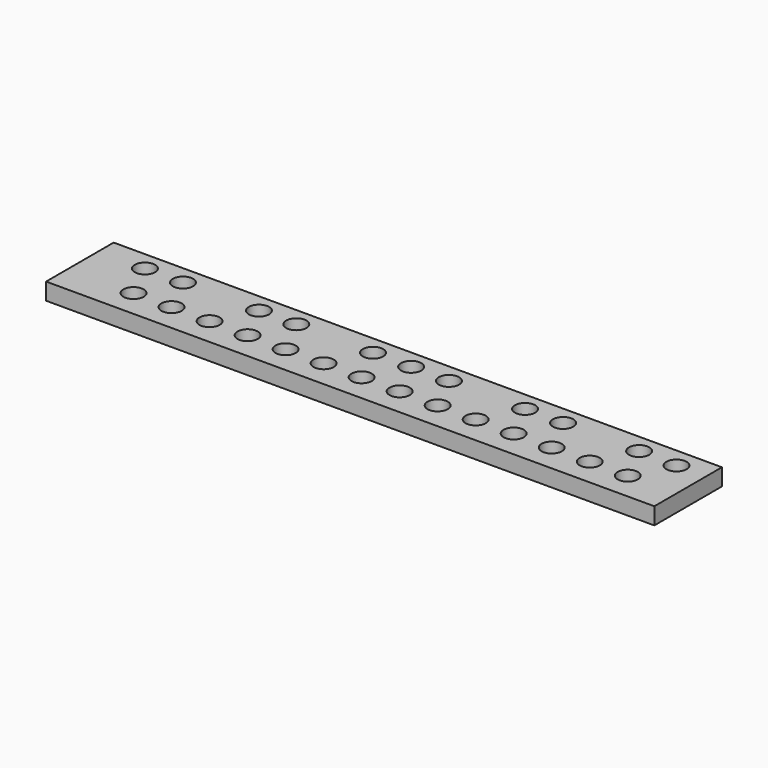
from build123d import *

# Parameters (mm, degrees)
F0_W     = 254
F0_H     = 50.8
F1_DEPTH = 1828.7999629974
F2_R     = 30.48
F3_DEPTH = 127


# Not quite as in the source:
# - a feature names something its author has since deleted; it is built from what else it names


with BuildPart() as f1:
    # F0 (on Right) → F1 (new body)
    with BuildSketch(Plane.YZ):
        with Locations((-10.6218170047, -93.1090038955)):
            Rectangle(F0_W, F0_H)
    extrude(amount=F1_DEPTH)

    # F2 (on Top) → F3 (cut)
    with BuildSketch(Plane.XY):
        with Locations((139.7, 59.2281829953)):
            Circle(F2_R)
        with Locations((254, 59.2281829953)):
            Circle(F2_R)
        with Locations((196.9066466086, -55.0718170047)):
            Circle(F2_R)
        with Locations((311.2066466086, -55.0718170047)):
            Circle(F2_R)
        with Locations((425.5066466086, -55.0718170047)):
            Circle(F2_R)
        with Locations((539.8066466086, -55.0718170047)):
            Circle(F2_R)
        with Locations((482.6, 59.2281829953)):
            Circle(F2_R)
        with Locations((594.391644001, 59.8655641079)):
            Circle(F2_R)
        with Locations((654.1066466086, -55.0718170047)):
            Circle(F2_R)
        with Locations((768.4066466086, -55.0718170047)):
            Circle(F2_R)
        with Locations((882.7066466086, -55.0718170047)):
            Circle(F2_R)
        with Locations((825.5, 59.2281829953)):
            Circle(F2_R)
        with Locations((940.1113390923, 59.2281829953)):
            Circle(F2_R)
        with Locations((997.0066466086, -55.0718170047)):
            Circle(F2_R)
        with Locations((1111.3066466086, -55.0718170047)):
            Circle(F2_R)
        with Locations((1054.1, 58.8000789285)):
            Circle(F2_R)
        with Locations((1225.6066466086, -55.0718170047)):
            Circle(F2_R)
        with Locations((1339.9066466086, -55.0718170047)):
            Circle(F2_R)
        with Locations((1282.7, 59.2281829953)):
            Circle(F2_R)
        with Locations((1397, 59.2281829953)):
            Circle(F2_R)
        with Locations((1454.2066466086, -55.0718170047)):
            Circle(F2_R)
        with Locations((1568.5066466086, -55.0718170047)):
            Circle(F2_R)
        with Locations((1625.6, 59.2281829953)):
            Circle(F2_R)
        with Locations((1682.8066466086, -55.0718170047)):
            Circle(F2_R)
        with Locations((1739.9, 56.6691346467)):
            Circle(F2_R)
    extrude(amount=-F3_DEPTH, mode=Mode.SUBTRACT)


solid = f1.part
